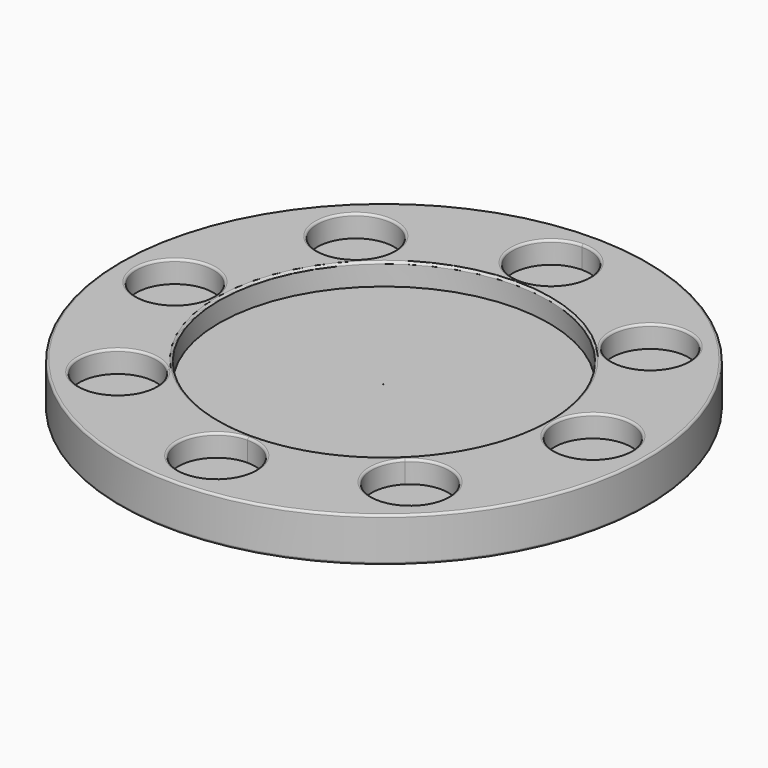
from build123d import *

# Parameters (mm, degrees)
F1_DEPTH = 50.8
F2_DEPTH = 25.4
F3_DEPTH = 25.4
F4_R     = 2.54


with BuildPart() as f1:
    # F0 (on Top) → F1 (new body)
    with BuildSketch(Plane.XY):
        with BuildLine():
            Line((285.75, 0), (304.8, 0))
            ThreePointArc((304.8, 0), (215.5261469057, 215.5261469057), (0, 304.8))
            Line((0, 304.8), (0, 285.75))
            ThreePointArc((0, 285.75), (31.4308964237, 272.7308964237), (44.45, 241.3))
            ThreePointArc((44.45, 241.3), (31.4308964237, 209.8691035763), (0, 196.85))
            Line((0, 196.85), (0, 190.5))
            ThreePointArc((0, 190.5), (73.853478682, 175.6015765492), (136.1552471412, 133.2366266306))
            ThreePointArc((136.1552471412, 133.2366266306), (176.3913611552, 71.9467699747), (190.5, 0))
            Line((190.5, 0), (196.85, 0))
            ThreePointArc((196.85, 0), (241.3, 44.45), (285.75, 0))
        make_face()
        with BuildLine():
            ThreePointArc((216.8510989977, 168.8299471788), (189.2247000531, 127.686673761), (140.6860169942, 137.6858293793))
            ThreePointArc((140.6860169942, 137.6858293793), (155.5774979423, 209.9732205965), (216.8510989977, 168.8299471788))
        make_face(mode=Mode.SUBTRACT)
        with BuildLine():
            ThreePointArc((0, -304.8), (215.5261469057, -215.5261469057), (304.8, 0))
            Line((304.8, 0), (285.75, 0))
            ThreePointArc((285.75, 0), (241.3, -44.45), (196.85, 0))
            Line((196.85, 0), (190.5, 0))
            ThreePointArc((190.5, 0), (175.4899748966, -74.1182751471), (132.825262879, -136.5565799994))
            ThreePointArc((132.825262879, -136.5565799994), (71.6806163133, -176.499686246), (0, -190.5))
            Line((0, -190.5), (0, -196.85))
            ThreePointArc((0, -196.85), (31.4308964237, -209.8691035763), (44.45, -241.3))
            ThreePointArc((44.45, -241.3), (31.4308964237, -272.7308964237), (0, -285.75))
            Line((0, -285.75), (0, -304.8))
        make_face()
        with BuildLine():
            ThreePointArc((212.8688597149, -172.8027132088), (151.2222544713, -213.791483233), (137.2747419154, -141.0876312053))
            ThreePointArc((137.2747419154, -141.0876312053), (185.6154649585, -131.8139431847), (212.8688597149, -172.8027132088))
        make_face(mode=Mode.SUBTRACT)
        with BuildLine():
            Line((0, 285.75), (0, 304.8))
            ThreePointArc((0, 304.8), (-215.5261469057, 215.5261469057), (-304.8, 0))
            Line((-304.8, 0), (-285.75, 0))
            ThreePointArc((-285.75, 0), (-241.3, 44.45), (-196.85, 0))
            Line((-196.85, 0), (-190.5, 0))
            ThreePointArc((-190.5, 0), (-175.8413413963, 73.2807795807), (-134.1212844519, 135.283890604))
            ThreePointArc((-134.1212844519, 135.283890604), (-72.5212687421, 176.1559410864), (0, 190.5))
            Line((0, 190.5), (0, 196.85))
            ThreePointArc((0, 196.85), (-44.45, 241.3), (0, 285.75))
        make_face()
        with BuildLine():
            ThreePointArc((-125.2648812879, 171.5300238135), (-128.7261112637, 154.3334185698), (-138.5707634883, 139.81494181))
            ThreePointArc((-138.5707634883, 139.81494181), (-210.703651312, 188.7266290571), (-125.2648812879, 171.5300238135))
        make_face(mode=Mode.SUBTRACT)
        with BuildLine():
            ThreePointArc((-304.8, 0), (-215.5261469057, -215.5261469057), (0, -304.8))
            Line((0, -304.8), (0, -285.75))
            ThreePointArc((0, -285.75), (-44.45, -241.3), (0, -196.85))
            Line((0, -196.85), (0, -190.5))
            ThreePointArc((0, -190.5), (-73.5459383628, -175.7306033403), (-135.6878962911, -133.7125454103))
            ThreePointArc((-135.6878962911, -133.7125454103), (-176.265133029, -72.2554695388), (-190.5, 0))
            Line((-190.5, 0), (-196.85, 0))
            ThreePointArc((-196.85, 0), (-241.3, -44.45), (-285.75, 0))
            Line((-285.75, 0), (-304.8, 0))
        make_face()
        with BuildLine():
            ThreePointArc((-127.4837481475, -169.3058659585), (-213.0770215653, -186.1294670139), (-140.218666144, -138.1617481589))
            ThreePointArc((-140.218666144, -138.1617481589), (-130.7904747298, -152.482264903), (-127.4837481475, -169.3058659585))
        make_face(mode=Mode.SUBTRACT)
    extrude(amount=F1_DEPTH)

    # F0 (on Top) → F2, piece 9 (join)
    with BuildSketch(Plane.XY):
        with BuildLine():
            Line((0.4759973175, 0), (190.5, 0))
            ThreePointArc((190.5, 0), (176.3913611552, 71.9467699747), (136.1552471412, 133.2366266306))
            Line((136.1552471412, 133.2366266306), (0.4759973175, 0))
        make_face()
        with BuildLine():
            ThreePointArc((132.825262879, -136.5565799994), (175.4899748966, -74.1182751471), (190.5, 0))
            Line((190.5, 0), (0.4759973175, 0))
            Line((0.4759973175, 0), (0, -0.467427974))
            Line((0, -0.467427974), (0, -1.296235447))
            Line((0, -1.296235447), (132.825262879, -136.5565799994))
        make_face()
        with BuildLine():
            Line((0, 0), (0, 190.5))
            ThreePointArc((0, 190.5), (-72.5212687421, 176.1559410864), (-134.1212844519, 135.283890604))
            Line((-134.1212844519, 135.283890604), (-1.2728994191, 0))
            Line((-1.2728994191, 0), (0, 0))
        make_face()
        with BuildLine():
            ThreePointArc((136.1552471412, 133.2366266306), (73.853478682, 175.6015765492), (0, 190.5))
            Line((0, 190.5), (0, 0))
            Line((0, 0), (0.4759973175, 0))
            Line((0.4759973175, 0), (136.1552471412, 133.2366266306))
        make_face()
        with BuildLine():
            Line((0, -1.296235447), (0, -190.5))
            ThreePointArc((0, -190.5), (71.6806163133, -176.499686246), (132.825262879, -136.5565799994))
            Line((132.825262879, -136.5565799994), (0, -1.296235447))
        make_face()
        with BuildLine():
            ThreePointArc((-135.6878962911, -133.7125454103), (-73.5459383628, -175.7306033403), (0, -190.5))
            Line((0, -190.5), (0, -1.296235447))
            Line((0, -1.296235447), (-0.4143353614, -0.8743040875))
            Line((-0.4143353614, -0.8743040875), (-135.6878962911, -133.7125454103))
        make_face()
        with BuildLine():
            Line((-1.2728994191, 0), (-190.5, 0))
            ThreePointArc((-190.5, 0), (-176.265133029, -72.2554695388), (-135.6878962911, -133.7125454103))
            Line((-135.6878962911, -133.7125454103), (-0.4143353614, -0.8743040875))
            Line((-0.4143353614, -0.8743040875), (-1.2728994191, 0))
        make_face()
        with BuildLine():
            ThreePointArc((-134.1212844519, 135.283890604), (-175.8413413963, 73.2807795807), (-190.5, 0))
            Line((-190.5, 0), (-1.2728994191, 0))
            Line((-1.2728994191, 0), (-134.1212844519, 135.283890604))
        make_face()
    extrude(amount=F2_DEPTH)

    # F0 (on Top) → F3 (join)
    with BuildSketch(Plane.XY):
        with BuildLine():
            Line((-1.2728994191, 0), (-190.5, 0))
            ThreePointArc((-190.5, 0), (-176.265133029, -72.2554695388), (-135.6878962911, -133.7125454103))
            Line((-135.6878962911, -133.7125454103), (-0.4143353614, -0.8743040875))
            Line((-0.4143353614, -0.8743040875), (-1.2728994191, 0))
        make_face()
        with BuildLine():
            ThreePointArc((-135.6878962911, -133.7125454103), (-73.5459383628, -175.7306033403), (0, -190.5))
            Line((0, -190.5), (0, -1.296235447))
            Line((0, -1.296235447), (-0.4143353614, -0.8743040875))
            Line((-0.4143353614, -0.8743040875), (-135.6878962911, -133.7125454103))
        make_face()
        with BuildLine():
            Line((0, -1.296235447), (0, -190.5))
            ThreePointArc((0, -190.5), (71.6806163133, -176.499686246), (132.825262879, -136.5565799994))
            Line((132.825262879, -136.5565799994), (0, -1.296235447))
        make_face()
        with BuildLine():
            ThreePointArc((132.825262879, -136.5565799994), (175.4899748966, -74.1182751471), (190.5, 0))
            Line((190.5, 0), (0.4759973175, 0))
            Line((0.4759973175, 0), (0, -0.467427974))
            Line((0, -0.467427974), (0, -1.296235447))
            Line((0, -1.296235447), (132.825262879, -136.5565799994))
        make_face()
        with BuildLine():
            Line((0.4759973175, 0), (190.5, 0))
            ThreePointArc((190.5, 0), (176.3913611552, 71.9467699747), (136.1552471412, 133.2366266306))
            Line((136.1552471412, 133.2366266306), (0.4759973175, 0))
        make_face()
        with BuildLine():
            ThreePointArc((136.1552471412, 133.2366266306), (73.853478682, 175.6015765492), (0, 190.5))
            Line((0, 190.5), (0, 0))
            Line((0, 0), (0.4759973175, 0))
            Line((0.4759973175, 0), (136.1552471412, 133.2366266306))
        make_face()
        with BuildLine():
            Line((0, 0), (0, 190.5))
            ThreePointArc((0, 190.5), (-72.5212687421, 176.1559410864), (-134.1212844519, 135.283890604))
            Line((-134.1212844519, 135.283890604), (-1.2728994191, 0))
            Line((-1.2728994191, 0), (0, 0))
        make_face()
        with BuildLine():
            ThreePointArc((-134.1212844519, 135.283890604), (-175.8413413963, 73.2807795807), (-190.5, 0))
            Line((-190.5, 0), (-1.2728994191, 0))
            Line((-1.2728994191, 0), (-134.1212844519, 135.283890604))
        make_face()
    extrude(amount=F3_DEPTH)

    # F4
    f4_edges = [f1.edges().sort_by_distance(p)[0] for p in [
        (196.85, 0, 50.8),
        (0, 285.75, 50.8),
        (0, -196.85, 50.8),
        (304.8, 0, 50.8),
        (-285.75, 0, 50.8),
        (0, 190.5, 50.8),
        (204.116181, 199.974065, 50.8),
        (199.562978, -204.517795, 50.8),
        (-214.164881, 171.530024, 50.8),
        (-203.64883, -200.449984, 50.8),
        (304.8, 0, 0),
    ]]
    fillet(f4_edges, radius=F4_R)


with BuildPart() as f2:
    # F0 (on Top) → F2 (new body)
    with BuildSketch(Plane.XY):
        with BuildLine():
            ThreePointArc((216.8510989977, 168.8299471788), (155.5774979423, 209.9732205965), (140.6860169942, 137.6858293793))
            ThreePointArc((140.6860169942, 137.6858293793), (189.2247000531, 127.686673761), (216.8510989977, 168.8299471788))
        make_face()
    extrude(amount=F2_DEPTH)


with BuildPart() as f2b:
    # F0 (on Top) → F2, piece 2 (new body)
    with BuildSketch(Plane.XY):
        with BuildLine():
            ThreePointArc((212.8688597149, -172.8027132088), (185.6154649585, -131.8139431847), (137.2747419154, -141.0876312053))
            ThreePointArc((137.2747419154, -141.0876312053), (151.2222544713, -213.791483233), (212.8688597149, -172.8027132088))
        make_face()
    extrude(amount=F2_DEPTH)


with BuildPart() as f2c:
    # F0 (on Top) → F2, piece 3 (new body)
    with BuildSketch(Plane.XY):
        with BuildLine():
            ThreePointArc((-125.2648812879, 171.5300238135), (-210.703651312, 188.7266290571), (-138.5707634883, 139.81494181))
            ThreePointArc((-138.5707634883, 139.81494181), (-128.7261112637, 154.3334185698), (-125.2648812879, 171.5300238135))
        make_face()
    extrude(amount=F2_DEPTH)


with BuildPart() as f2d:
    # F0 (on Top) → F2, piece 4 (new body)
    with BuildSketch(Plane.XY):
        with BuildLine():
            ThreePointArc((-127.4837481475, -169.3058659585), (-130.7904747298, -152.482264903), (-140.218666144, -138.1617481589))
            ThreePointArc((-140.218666144, -138.1617481589), (-213.0770215653, -186.1294670139), (-127.4837481475, -169.3058659585))
        make_face()
    extrude(amount=F2_DEPTH)


with BuildPart() as f2e:
    # F0 (on Top) → F2, piece 5 (new body)
    with BuildSketch(Plane.XY):
        with BuildLine():
            Line((241.3, 0), (285.75, 0))
            ThreePointArc((285.75, 0), (241.3, 44.45), (196.85, 0))
            Line((196.85, 0), (241.3, 0))
        make_face()
        with BuildLine():
            ThreePointArc((196.85, 0), (241.3, -44.45), (285.75, 0))
            Line((285.75, 0), (241.3, 0))
            Line((241.3, 0), (196.85, 0))
        make_face()
    extrude(amount=F2_DEPTH)


with BuildPart() as f2f:
    # F0 (on Top) → F2, piece 6 (new body)
    with BuildSketch(Plane.XY):
        with BuildLine():
            Line((0, 241.3), (0, 285.75))
            ThreePointArc((0, 285.75), (-44.45, 241.3), (0, 196.85))
            Line((0, 196.85), (0, 241.3))
        make_face()
        with BuildLine():
            ThreePointArc((44.45, 241.3), (31.4308964237, 272.7308964237), (0, 285.75))
            Line((0, 285.75), (0, 241.3))
            Line((0, 241.3), (0, 196.85))
            ThreePointArc((0, 196.85), (31.4308964237, 209.8691035763), (44.45, 241.3))
        make_face()
    extrude(amount=F2_DEPTH)


with BuildPart() as f2g:
    # F0 (on Top) → F2, piece 7 (new body)
    with BuildSketch(Plane.XY):
        with BuildLine():
            Line((0, -241.3), (0, -285.75))
            ThreePointArc((0, -285.75), (31.4308964237, -272.7308964237), (44.45, -241.3))
            ThreePointArc((44.45, -241.3), (31.4308964237, -209.8691035763), (0, -196.85))
            Line((0, -196.85), (0, -241.3))
        make_face()
        with BuildLine():
            ThreePointArc((0, -196.85), (-44.45, -241.3), (0, -285.75))
            Line((0, -285.75), (0, -241.3))
            Line((0, -241.3), (0, -196.85))
        make_face()
    extrude(amount=F2_DEPTH)


with BuildPart() as f2h:
    # F0 (on Top) → F2, piece 8 (new body)
    with BuildSketch(Plane.XY):
        with BuildLine():
            Line((-241.3, 0), (-285.75, 0))
            ThreePointArc((-285.75, 0), (-241.3, -44.45), (-196.85, 0))
            Line((-196.85, 0), (-241.3, 0))
        make_face()
        with BuildLine():
            ThreePointArc((-196.85, 0), (-241.3, 44.45), (-285.75, 0))
            Line((-285.75, 0), (-241.3, 0))
            Line((-241.3, 0), (-196.85, 0))
        make_face()
    extrude(amount=F2_DEPTH)


solid = Compound([f1.part, f2.part, f2b.part, f2c.part, f2d.part, f2e.part, f2f.part, f2g.part, f2h.part])
